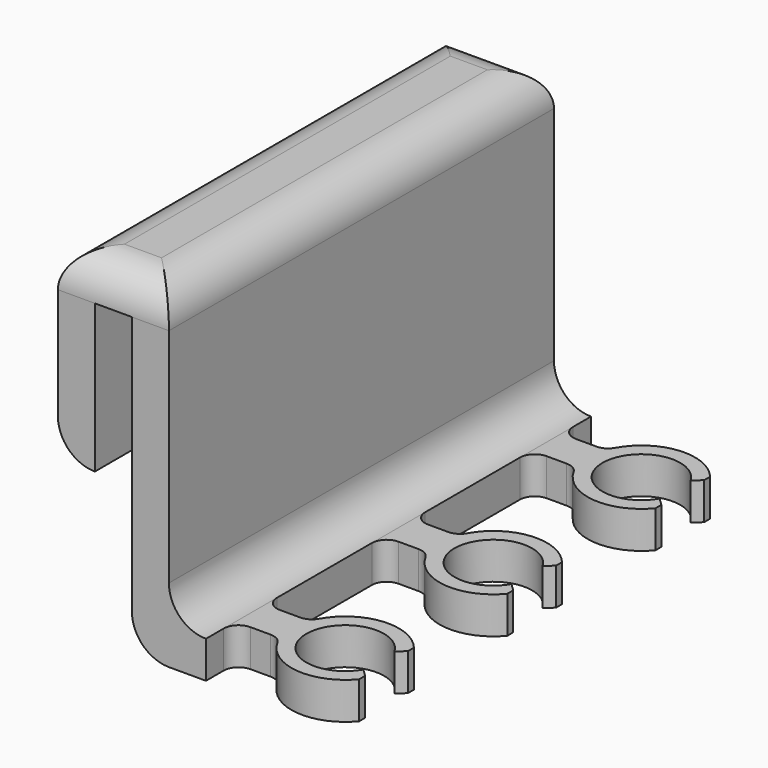
from build123d import *

# Parameters (mm, degrees)
F1_DEPTH = 5
F2_W     = 5
F2_H     = 65
F3_DEPTH = 40
F4_W     = 65
F4_H     = 5
F5_DEPTH = 5
F6_W     = 5
F6_H     = 65
F7_DEPTH = 25
F8_R     = 4.99999


# Not quite as in the source:
# - a fillet or chamfer is up to 0.001 mm smaller than in the source, because OpenCascade refuses the exact size


with BuildPart() as f1:
    # F0 (on Top) → F1 (new body)
    with BuildSketch(Plane.XY):
        with BuildLine():
            ThreePointArc((4.5503406659, -2.6185682776), (-5.25, 0), (4.5503406659, 2.6185682776))
            Line((4.5503406659, 2.6185682776), (5.5884995361, 3.6185682776))
            Line((5.5884995361, 3.6185682776), (5.5884995361, 4.6185682776))
            ThreePointArc((5.5884995361, 4.6185682776), (-0.6609820827, 7.2198062776), (-6.3342387349, 3.527027027))
            ThreePointArc((-6.3342387349, 3.527027027), (-7.0681915182, 2.7757688748), (-8.0816149376, 2.5))
            Line((-8.0816149376, 2.5), (-10.8053287944, 2.5))
            ThreePointArc((-10.8053287944, 2.5), (-12.2195423568, 3.0857864376), (-12.8053287944, 4.5))
            Line((-12.8053287944, 4.5), (-12.8053287944, 20.5))
            ThreePointArc((-12.8053287944, 20.5), (-12.2195423568, 21.9142135624), (-10.8053287944, 22.5))
            Line((-10.8053287944, 22.5), (-8.0816149376, 22.5))
            ThreePointArc((-8.0816149376, 22.5), (-7.0681915182, 22.2242311252), (-6.3342387349, 21.472972973))
            ThreePointArc((-6.3342387349, 21.472972973), (-0.6609820827, 17.7801937224), (5.5884995361, 20.3814317224))
            Line((5.5884995361, 20.3814317224), (5.5884995361, 21.3814317224))
            Line((5.5884995361, 21.3814317224), (4.5503406659, 22.3814317224))
            ThreePointArc((4.5503406659, 22.3814317224), (-5.25, 25), (4.5503406659, 27.6185682776))
            Line((4.5503406659, 27.6185682776), (5.5884995361, 28.6185682776))
            Line((5.5884995361, 28.6185682776), (5.5884995361, 29.6185682776))
            ThreePointArc((5.5884995361, 29.6185682776), (-0.6609820827, 32.2198062776), (-6.3342387349, 28.527027027))
            ThreePointArc((-6.3342387349, 28.527027027), (-7.0681915182, 27.7757688748), (-8.0816149376, 27.5))
            Line((-8.0816149376, 27.5), (-10.8053287944, 27.5))
            ThreePointArc((-10.8053287944, 27.5), (-12.2195423568, 28.0857864376), (-12.8053287944, 29.5))
            Line((-12.8053287944, 29.5), (-12.8053287944, 45.5))
            ThreePointArc((-12.8053287944, 45.5), (-12.2195423568, 46.9142135624), (-10.8053287944, 47.5))
            Line((-10.8053287944, 47.5), (-8.0816149376, 47.5))
            ThreePointArc((-8.0816149376, 47.5), (-7.0681915182, 47.2242311252), (-6.3342387349, 46.472972973))
            ThreePointArc((-6.3342387349, 46.472972973), (-0.6609820827, 42.7801937224), (5.5884995361, 45.3814317224))
            Line((5.5884995361, 45.3814317224), (5.5884995361, 46.3814317224))
            Line((5.5884995361, 46.3814317224), (4.5503406659, 47.3814317224))
            ThreePointArc((4.5503406659, 47.3814317224), (-5.25, 50), (4.5503406659, 52.6185682776))
            Line((4.5503406659, 52.6185682776), (5.5884995361, 53.6185682776))
            Line((5.5884995361, 53.6185682776), (5.5884995361, 54.6185682776))
            ThreePointArc((5.5884995361, 54.6185682776), (-0.6609820827, 57.2198062776), (-6.3342387349, 53.527027027))
            ThreePointArc((-6.3342387349, 53.527027027), (-7.0681915182, 52.7757688748), (-8.0816149376, 52.5))
            Line((-8.0816149376, 52.5), (-10.8053287944, 52.5))
            ThreePointArc((-10.8053287944, 52.5), (-12.2195423568, 53.0857864376), (-12.8053287944, 54.5))
            Line((-12.8053287944, 54.5), (-12.8053287944, 57.5))
            Line((-12.8053287944, 57.5), (-22.8053287944, 57.5))
            Line((-22.8053287944, 57.5), (-22.8053287944, -7.5))
            Line((-22.8053287944, -7.5), (-12.8053287944, -7.5))
            Line((-12.8053287944, -7.5), (-12.8053287944, -4.5))
            ThreePointArc((-12.8053287944, -4.5), (-12.2195423568, -3.0857864376), (-10.8053287944, -2.5))
            Line((-10.8053287944, -2.5), (-8.0816149376, -2.5))
            ThreePointArc((-8.0816149376, -2.5), (-7.0681915182, -2.7757688748), (-6.3342387349, -3.527027027))
            ThreePointArc((-6.3342387349, -3.527027027), (-0.6609820827, -7.2198062776), (5.5884995361, -4.6185682776))
            Line((5.5884995361, -4.6185682776), (5.5884995361, -3.6185682776))
            Line((5.5884995361, -3.6185682776), (4.5503406659, -2.6185682776))
        make_face()
    extrude(amount=F1_DEPTH)

    # F2 (on face) → F3 (join)
    with BuildSketch(Plane.XY.offset(5)):
        with Locations((-20.3053287944, 25)):
            Rectangle(F2_W, F2_H)
    extrude(amount=F3_DEPTH)

    # F4 (on face) → F5 (join)
    with BuildSketch(Plane(origin=(-22.8053287944, 0, 0), x_dir=(0, -1, 0), z_dir=(-1, 0, 0))):
        with Locations((-25, 42.5)):
            Rectangle(F4_W, F4_H)
    extrude(amount=F5_DEPTH)

    # F6 (on face) → F7 (join)
    with BuildSketch(Plane.XY.offset(45)):
        with Locations((-30.3053287944, 25)):
            Rectangle(F6_W, F6_H)
    extrude(amount=-F7_DEPTH)

    # F8 (radius 5 in the source; OpenCascade refuses exactly that, so slightly less here)
    f8_edges = [f1.edges().sort_by_distance(p)[0] for p in [
        (-32.805329, 25, 45),
        (-25.305329, -7.5, 45),
        (-17.805329, 25, 45),
        (-25.305329, 57.5, 45),
        (-17.805329, 25, 5),
        (-22.805329, 25, 0),
        (-32.805329, 25, 20),
    ]]
    fillet(f8_edges, radius=F8_R)


solid = f1.part
